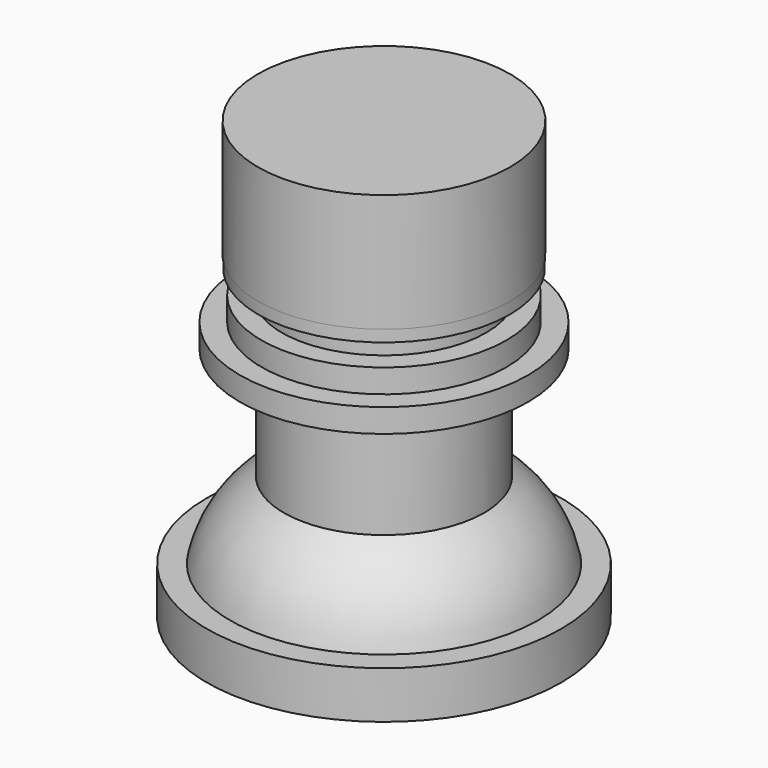
from build123d import *

# Parameters (mm, degrees)
F0_R      = 19.0458801966
F2_DEPTH  = 5.08
F1_R      = 16.5564413769
F3_DEPTH  = 15.24
F5_R      = 10.7565912882
F6_DEPTH  = 25.4
F7_R      = 15.4966869389
F8_DEPTH  = 2.54
F9_R      = 13.1720463189
F10_DEPTH = 2.54
F11_R     = 10.9761291002
F12_DEPTH = 2.54
F13_R     = 13.5071591259
F14_DEPTH = 1.27
F15_R     = 13.5553537987
F16_DEPTH = 12.7


# Not quite as in the source:
# - a fillet or chamfer that OpenCascade refuses, or shapes differently, is made with other operations: its cross-section is extruded or revolved along the edge and cut away or added


with BuildPart() as f2:
    # F0 (on Top) → F2 (new body)
    with BuildSketch(Plane.XY):
        Circle(F0_R)
    extrude(amount=F2_DEPTH)

    # F1 (on Top) → F3 (join)
    with BuildSketch(Plane.XY):
        Circle(F1_R)
    extrude(amount=F3_DEPTH)

    # F4: fillet of radius 12.7 on 1 edges, made by hand

    # F4_s1 → F4_t2 (revolve, cut)
    with BuildSketch(Plane.XZ):
        with BuildLine():
            ThreePointArc((16.5564413769, 5.08), (12.1452187403, 12.3773776994), (4.1130334835, 15.24))
            Line((4.1130334835, 15.24), (16.5564413769, 15.24))
            Line((16.5564413769, 15.24), (16.5564413769, 5.08))
        make_face()
    revolve(axis=Axis((0, 0, 15.24), (0, 0, 1)), mode=Mode.SUBTRACT)

    # F5 (on Top) → F6 (join)
    with BuildSketch(Plane.XY):
        Circle(F5_R)
    extrude(amount=F6_DEPTH)

    # F7 (on face) → F8 (join)
    with BuildSketch(Plane.XY.offset(25.4)):
        Circle(F7_R)
    extrude(amount=F8_DEPTH)

    # F9 (on face) → F10 (join)
    with BuildSketch(Plane.XY.offset(27.94)):
        Circle(F9_R)
    extrude(amount=F10_DEPTH)

    # F11 (on face) → F12 (join)
    with BuildSketch(Plane.XY.offset(30.48)):
        Circle(F11_R)
    extrude(amount=F12_DEPTH)

    # F13 (on face) → F14 (join)
    with BuildSketch(Plane.XY.offset(33.02)):
        Circle(F13_R)
    extrude(amount=F14_DEPTH)

    # F15 (on face) → F16 (join)
    with BuildSketch(Plane.XY.offset(34.29)):
        Circle(F15_R)
    extrude(amount=F16_DEPTH)


solid = f2.part
